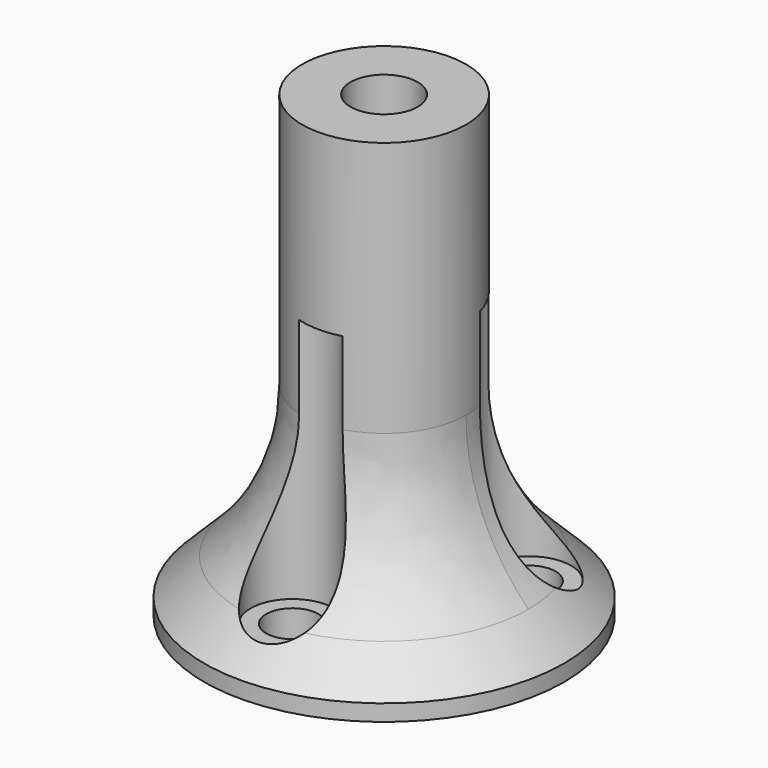
from build123d import *

# Parameters (mm, degrees)
F0_R        = 13
F1_DEPTH    = 6
F2_R        = 5
F3_DEPTH    = 21
F4_S5_R     = 5
F4_T6_DEPTH = 20
F5_R        = 13
F6_DEPTH    = 1
F8_R        = 1.6
F9_DEPTH    = 25
F10_R       = 2.55
F11_DEPTH   = 15
F12_R       = 2.05
F13_DEPTH   = 30


# Not quite as in the source:
# - a fillet or chamfer that OpenCascade refuses, or shapes differently, is made with other operations: its cross-section is extruded or revolved along the edge and cut away or added


with BuildPart() as f1:
    # F0 (on Top) → F1 (new body)
    with BuildSketch(Plane.XY):
        Circle(F0_R)
    extrude(amount=F1_DEPTH)

    # F2 (on face) → F3 (join)
    with BuildSketch(Plane.XY.offset(6)):
        Circle(F2_R)
    extrude(amount=F3_DEPTH)

    # F4: chamfer of 8 on 1 edges, made by hand


with BuildPart() as f4_tool2:
    # F4_s3 → F4_t4 (revolve)
    with BuildSketch(Plane.XZ):
        Polygon((13, -2), (5, 6), (13, 6), align=None)
    revolve(axis=Axis((0, 0, 6), (0, 0, 1)))

    # F4_s5 → F4_t6 (cut, symmetric)
    with BuildSketch(Plane.XY.offset(2)):
        Circle(F4_S5_R)
    extrude(amount=F4_T6_DEPTH, both=True, mode=Mode.SUBTRACT)


with BuildPart() as f1_1:
    add(f1.part)

    # F4_t1: cut F4_tool2
    add(f4_tool2.part, mode=Mode.SUBTRACT)

    # F5
    f5_edges = [f1_1.edges().sort_by_distance(p)[0] for p in [
        (-5, 0, 6),
    ]]
    fillet(f5_edges, radius=F5_R)

    # F6 (add): a face of the model
    f6_faces = [f1_1.faces().sort_by_distance(p)[0] for p in [
        (0, 0, 0),
    ]]
    extrude(f6_faces, amount=F6_DEPTH)

    # F8 (on offset) → F9 (cut)
    with BuildSketch(Plane(origin=(0, 0, 1.4), x_dir=(1, 0, 0), z_dir=(0, 0, -1))):
        with Locations((6.0621778265, -3.5)):
            Circle(F8_R)
        with Locations((0, 7)):
            Circle(F8_R)
        with Locations((-6.0621778265, -3.5)):
            Circle(F8_R)
    extrude(amount=F9_DEPTH, mode=Mode.SUBTRACT)

    # F10 (on offset) → F11 (cut)
    with BuildSketch(Plane(origin=(0, 0, 1.4), x_dir=(1, 0, 0), z_dir=(0, 0, -1))):
        with Locations((0, 7)):
            Circle(F10_R)
        with Locations((6.0621778265, -3.5)):
            Circle(F10_R)
        with Locations((-6.0621778265, -3.5)):
            Circle(F10_R)
    extrude(amount=-F11_DEPTH, mode=Mode.SUBTRACT)

    # F12 (on face) → F13 (cut)
    with BuildSketch(Plane.XY.offset(27)):
        Circle(F12_R)
    extrude(amount=-F13_DEPTH, mode=Mode.SUBTRACT)


solid = f1_1.part
